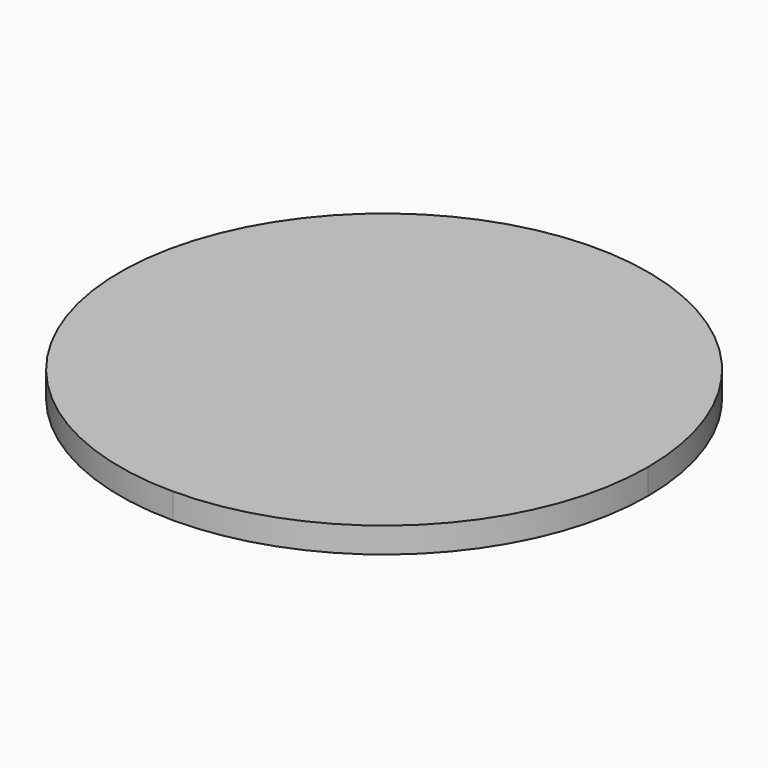
from build123d import *

# Parameters (mm, degrees)
F1_DEPTH = 3.175


# Not quite as in the source:
# - the program builds the solid bodies; features that only make, move or delete a surface that nothing else refers to are left out


with BuildPart() as f1:
    # F0 (on Top) → F1 (new body)
    with BuildSketch(Plane.XY):
        with BuildLine():
            ThreePointArc((0, -32.8952459435), (23.2604514755, -23.2604514755), (32.8952459435, 0))
            ThreePointArc((32.8952459435, 0), (-23.2604514755, 23.2604514755), (0, -32.8952459435))
        make_face()
    extrude(amount=F1_DEPTH)


solid = f1.part
